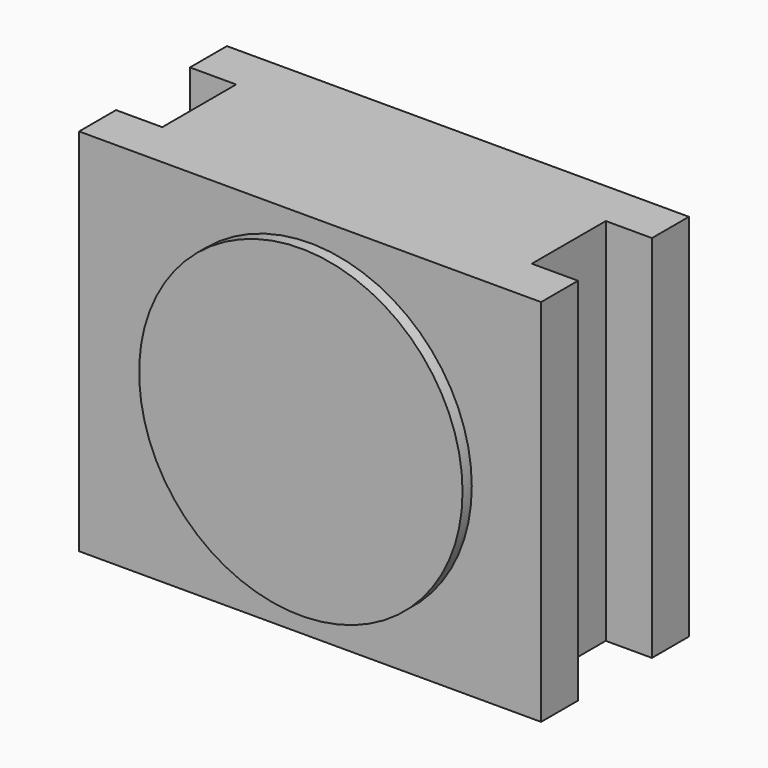
from build123d import *

# Parameters (mm, degrees)
F0_W     = 50.8
F0_H     = 50.8
F1_DEPTH = 12.7
F2_W     = 6.35
F2_H     = 50.8
F2_W_2   = 50.8
F3_DEPTH = 6.35
F4_W     = 6.35
F4_H     = 50.8
F4_W_2   = 50.8
F5_DEPTH = 6.35
F6_R     = 9.525
F7_DEPTH = 38.1
F8_R     = 22.225
F8_R_2   = 9.525
F9_DEPTH = 1.5875


# Not quite as in the source:
# - a feature names something its author has since deleted; it is built from what else it names


with BuildPart() as f1:
    # F0 (on Front) → F1 (new body)
    with BuildSketch(Plane.XZ):
        Rectangle(F0_W, F0_H)
    extrude(amount=F1_DEPTH)

    # F2 (on face) → F3 (join)
    with BuildSketch(Plane.XZ.offset(12.7)):
        with Locations((-28.575, 0)):
            Rectangle(F2_W, F2_H)
        Rectangle(F2_W_2, F2_H)
        with Locations((28.575, 0)):
            Rectangle(F2_W, F2_H)
    extrude(amount=F3_DEPTH)

    # F4 (on face) → F5 (join)
    with BuildSketch(Plane(origin=(0, 0, 0), x_dir=(-1, 0, 0), z_dir=(0, 1, 0))):
        with Locations((28.575, 0)):
            Rectangle(F4_W, F4_H)
        Rectangle(F4_W_2, F4_H)
        with Locations((-28.575, 0)):
            Rectangle(F4_W, F4_H)
    extrude(amount=F5_DEPTH)

    # F6 (on face) → F7 (cut)
    with BuildSketch(Plane.XZ.offset(19.05)):
        Circle(F6_R)
    extrude(amount=-F7_DEPTH, mode=Mode.SUBTRACT)

    # F8 (on face) → F9 (join)
    with BuildSketch(Plane.XZ.offset(19.05)):
        Circle(F8_R)
        Circle(F8_R_2, mode=Mode.SUBTRACT)
        Circle(F8_R_2)
    extrude(amount=F9_DEPTH)


solid = f1.part
